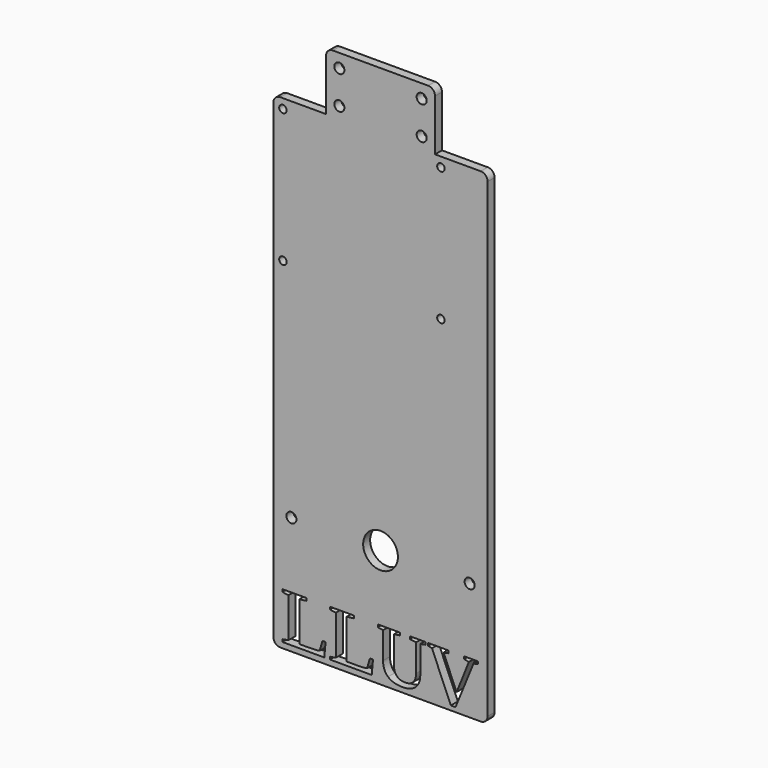
from build123d import *

# Parameters (mm, degrees)
F0_R     = 1.85
F0_R_2   = 6.375
F0_R_3   = 1.3716
F1_DEPTH = 3.2004


with BuildPart() as f1:
    # F0 (on Front) → F1 (new body)
    with BuildSketch(Plane.XZ):
        with BuildLine():
            ThreePointArc((-79.689629, -272.1204697257), (-78.9456802243, -273.91652095), (-77.149629, -274.6604697257))
            Line((-77.149629, -274.6604697257), (-3.589629, -274.6604697257))
            ThreePointArc((-3.589629, -274.6604697257), (-1.7935777758, -273.9165209499), (-1.049629, -272.1204697257))
            Line((-1.049629, -272.1204697257), (-1.049629, -99.4004697257))
            ThreePointArc((-1.049629, -99.4004697257), (-1.7935777758, -97.6044185016), (-3.589629, -96.8604697257))
            Line((-3.589629, -96.8604697257), (-20.354629, -96.8604697257))
            Line((-20.354629, -96.8604697257), (-20.354629, -78.0314697257))
            ThreePointArc((-20.354629, -78.0314697257), (-21.0985777758, -76.2354185016), (-22.894629, -75.4914697257))
            Line((-22.894629, -75.4914697257), (-57.844629, -75.4914697257))
            ThreePointArc((-57.844629, -75.4914697257), (-59.6406802243, -76.2354185015), (-60.384629, -78.0314697257))
            Line((-60.384629, -78.0314697257), (-60.384629, -96.8604697257))
            Line((-60.384629, -96.8604697257), (-77.149629, -96.8604697257))
            ThreePointArc((-77.149629, -96.8604697257), (-78.9456802243, -97.6044185015), (-79.689629, -99.4004697257))
            Line((-79.689629, -99.4004697257), (-79.689629, -272.1204697257))
        make_face()
        with BuildLine():
            Line((-67.5448753625, -255.545025575), (-67.5448753625, -256.4746303251))
            Line((-67.5448753625, -256.4746303251), (-70.1828327017, -256.808961858))
            Line((-70.1828327017, -256.808961858), (-70.1828327017, -271.2830709061))
            Line((-70.1828327017, -271.2830709061), (-66.7049693163, -271.2830709061))
            add(Edge.make_bspline(
                [(-66.7049693163, -271.2830709061), (-63.9895449146, -271.2830709061), (-62.7133769901, -271.0262064356)],
                knots=[0, 0, 0, 1, 1, 1], degree=2))
            Line((-62.7133769901, -271.0262064356), (-61.6696102531, -267.4708759878))
            Line((-61.6696102531, -267.4708759878), (-60.5239131707, -267.4708759878))
            Line((-60.5239131707, -267.4708759878), (-61.0091016149, -272.6326286793))
            Line((-61.0091016149, -272.6326286793), (-76.3883521301, -272.6326286793))
            Line((-76.3883521301, -272.6326286793), (-76.3883521301, -271.7030239291))
            Line((-76.3883521301, -271.7030239291), (-74.1948110969, -271.3564607548))
            Line((-74.1948110969, -271.3564607548), (-74.1948110969, -256.808961858))
            Line((-74.1948110969, -256.808961858), (-76.3720432749, -256.4746303251))
            Line((-76.3720432749, -256.4746303251), (-76.3720432749, -255.545025575))
            Line((-76.3720432749, -255.545025575), (-67.5448753625, -255.545025575))
        make_face(mode=Mode.SUBTRACT)
        with Locations((-73.079629, -231.3779697257)):
            Circle(F0_R, mode=Mode.SUBTRACT)
        with BuildLine():
            Line((-50.1392495805, -255.545025575), (-50.1392495805, -256.4746303251))
            Line((-50.1392495805, -256.4746303251), (-52.7772069197, -256.808961858))
            Line((-52.7772069197, -256.808961858), (-52.7772069197, -271.2830709061))
            Line((-52.7772069197, -271.2830709061), (-49.2993435343, -271.2830709061))
            add(Edge.make_bspline(
                [(-49.2993435343, -271.2830709061), (-46.5839191327, -271.2830709061), (-45.3077512081, -271.0262064356)],
                knots=[0, 0, 0, 1, 1, 1], degree=2))
            Line((-45.3077512081, -271.0262064356), (-44.2639844712, -267.4708759878))
            Line((-44.2639844712, -267.4708759878), (-43.1182873888, -267.4708759878))
            Line((-43.1182873888, -267.4708759878), (-43.6034758329, -272.6326286793))
            Line((-43.6034758329, -272.6326286793), (-58.9827263482, -272.6326286793))
            Line((-58.9827263482, -272.6326286793), (-58.9827263482, -271.7030239291))
            Line((-58.9827263482, -271.7030239291), (-56.789185315, -271.3564607548))
            Line((-56.789185315, -271.3564607548), (-56.789185315, -256.808961858))
            Line((-56.789185315, -256.808961858), (-58.9664174929, -256.4746303251))
            Line((-58.9664174929, -256.4746303251), (-58.9664174929, -255.545025575))
            Line((-58.9664174929, -255.545025575), (-50.1392495805, -255.545025575))
        make_face(mode=Mode.SUBTRACT)
        with BuildLine():
            add(Edge.make_bspline(
                [(-34.3828567872, -269.9824396987), (-33.345205871, -271.0792102152), (-31.3432938872, -271.0792102152)],
                knots=[0, 0, 0, 1, 1, 1], degree=2))
            add(Edge.make_bspline(
                [(-31.3432938872, -271.0792102152), (-29.4310806073, -271.0792102152), (-28.3873138703, -270.0089415885)],
                knots=[0, 0, 0, 1, 1, 1], degree=2))
            add(Edge.make_bspline(
                [(-28.3873138703, -270.0089415885), (-27.3435471333, -268.9386729617), (-27.3435471333, -266.8592939153)],
                knots=[0, 0, 0, 1, 1, 1], degree=2))
            Line((-27.3435471333, -266.8592939153), (-27.3435471333, -256.808961858))
            Line((-27.3435471333, -256.808961858), (-29.6349412981, -256.4746303251))
            Line((-29.6349412981, -256.4746303251), (-29.6349412981, -255.545025575))
            Line((-29.6349412981, -255.545025575), (-23.8249116098, -255.545025575))
            Line((-23.8249116098, -255.545025575), (-23.8249116098, -256.4746303251))
            Line((-23.8249116098, -256.4746303251), (-25.7615881726, -256.808961858))
            Line((-25.7615881726, -256.808961858), (-25.7615881726, -266.7573635699))
            add(Edge.make_bspline(
                [(-25.7615881726, -266.7573635699), (-25.7615881726, -269.7133435868), (-27.4699407616, -271.2932639406)],
                knots=[0, 0, 0, 1, 1, 1], degree=2))
            add(Edge.make_bspline(
                [(-27.4699407616, -271.2932639406), (-29.1782933507, -272.8731842944), (-32.3503656998, -272.8731842944)],
                knots=[0, 0, 0, 1, 1, 1], degree=2))
            add(Edge.make_bspline(
                [(-32.3503656998, -272.8731842944), (-35.7793025193, -272.8731842944), (-37.607932916, -271.2749164784)],
                knots=[0, 0, 0, 1, 1, 1], degree=2))
            add(Edge.make_bspline(
                [(-37.607932916, -271.2749164784), (-39.4365633126, -269.6766486624), (-39.4365633126, -266.6554332245)],
                knots=[0, 0, 0, 1, 1, 1], degree=2))
            Line((-39.4365633126, -266.6554332245), (-39.4365633126, -256.808961858))
            Line((-39.4365633126, -256.808961858), (-41.3732398754, -256.4746303251))
            Line((-41.3732398754, -256.4746303251), (-41.3732398754, -255.545025575))
            Line((-41.3732398754, -255.545025575), (-33.2310438841, -255.545025575))
            Line((-33.2310438841, -255.545025575), (-33.2310438841, -256.4746303251))
            Line((-33.2310438841, -256.4746303251), (-35.4205077035, -256.808961858))
            Line((-35.4205077035, -256.808961858), (-35.4205077035, -266.8348306324))
            add(Edge.make_bspline(
                [(-35.4205077035, -266.8348306324), (-35.4205077035, -268.8856691821), (-34.3828567872, -269.9824396987)],
                knots=[0, 0, 0, 1, 1, 1], degree=2))
        make_face(mode=Mode.SUBTRACT)
        with Locations((-40.364429, -231.3788697257)):
            Circle(F0_R_2, mode=Mode.SUBTRACT)
        Polygon((-9.656593598, -255.545025575), (-4.6253117486, -255.545025575), (-4.6253117486, -256.4746303251), (-6.2439656337, -256.8211934995), (-12.8449748024, -273.0281184195), (-14.5370185362, -273.0281184195), (-21.4805136654, -256.8211934995), (-22.8830752182, -256.4746303251), (-22.8830752182, -255.545025575), (-15.4543916449, -255.545025575), (-15.4543916449, -256.4746303251), (-17.227979655, -256.8211934995), (-12.4209445655, -268.021299853), (-7.9360093675, -256.8211934995), (-9.656593598, -256.4746303251), align=None, mode=Mode.SUBTRACT)
        with Locations((-7.659629, -231.3779697257)):
            Circle(F0_R, mode=Mode.SUBTRACT)
        with Locations((-76.184429, -149.3622697257)):
            Circle(F0_R_3, mode=Mode.SUBTRACT)
        with Locations((-76.184429, -100.3656697257)):
            Circle(F0_R_3, mode=Mode.SUBTRACT)
        with Locations((-55.482429, -92.6280697257)):
            Circle(F0_R, mode=Mode.SUBTRACT)
        with Locations((-55.482429, -80.4614697257)):
            Circle(F0_R, mode=Mode.SUBTRACT)
        with Locations((-18.196229, -149.3622697257)):
            Circle(F0_R_3, mode=Mode.SUBTRACT)
        with Locations((-25.256829, -92.6280697257)):
            Circle(F0_R, mode=Mode.SUBTRACT)
        with Locations((-25.256829, -80.4614697257)):
            Circle(F0_R, mode=Mode.SUBTRACT)
        with Locations((-18.196229, -100.3656697257)):
            Circle(F0_R_3, mode=Mode.SUBTRACT)
    extrude(amount=F1_DEPTH)


solid = f1.part
